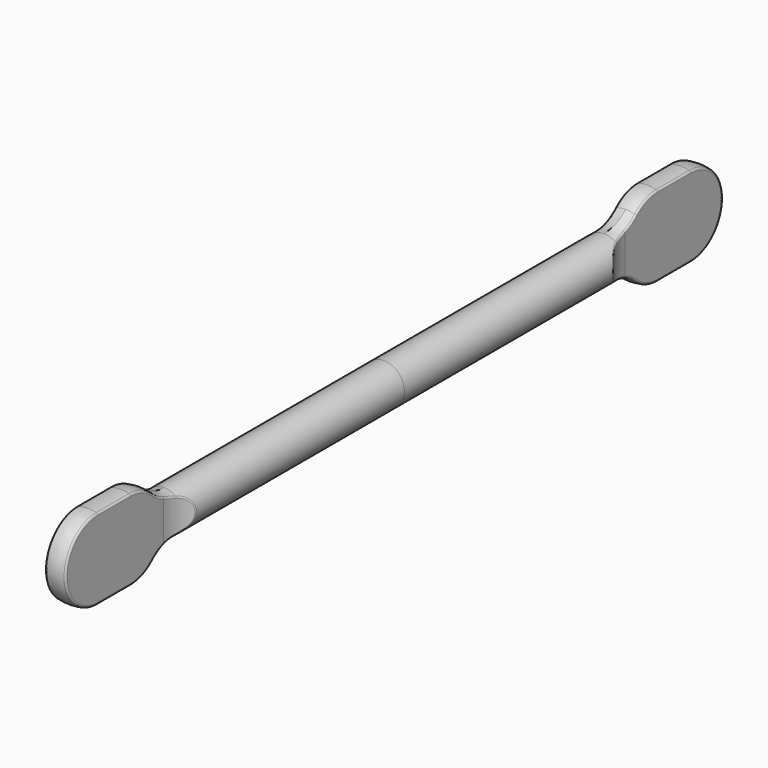
from build123d import *

# Parameters (mm, degrees)
F2_R          = 5
F4_DEPTH      = 5.001
F4_DEPTH_BACK = 5.001
F7_R          = 0.25


with BuildPart() as f1:
    # F0 (on Right) → F1 (revolve)
    with BuildSketch(Plane.YZ):
        with BuildLine():
            Line((35.6698729811, 2.5), (0, 2.5))
            Line((0, 2.5), (0, 0))
            Line((0, 0), (50, 0))
            ThreePointArc((50, 0), (48.5355339059, 3.5355339059), (45, 5))
            Line((45, 5), (40, 5))
            ThreePointArc((40, 5), (37.5, 4.3301270189), (35.6698729811, 2.5))
        make_face()
    revolve(axis=Axis((0, 25, 0), (0, -1, 0)))

    # F2
    f2_edges = [f1.edges().sort_by_distance(p)[0] for p in [
        (0, 35.669873, -2.5),
    ]]
    fillet(f2_edges, radius=F2_R)


with BuildPart() as f4:
    # F3 (on Top) → F4 (new body, two sides)
    with BuildSketch(Plane.XY) as f4_sk:
        with BuildLine():
            Line((-25, 75), (-25, 30))
            Line((-25, 30), (-6.25, 30))
            ThreePointArc((-6.25, 30), (-2.7144660941, 31.4644660941), (-1.25, 35))
            Line((-1.25, 35), (-1.25, 75))
            Line((-1.25, 75), (-25, 75))
        make_face()
    extrude(amount=-F4_DEPTH)
    extrude(f4_sk.sketch, amount=F4_DEPTH_BACK)


with BuildPart() as f5_1:
    # F5: instance of F4
    add(f4.part.mirror(Plane.YZ))


with BuildPart() as f1_1:
    add(f1.part)

    # F6: cut F4, F5_1
    add(f4.part, mode=Mode.SUBTRACT)
    add(f5_1.part, mode=Mode.SUBTRACT)

    # F7
    f7_edges = [f1_1.edges().sort_by_distance(p)[0] for p in [
        (-1.25, 49.841229, 0),
        (1.25, 49.841229, 0),
    ]]
    fillet(f7_edges, radius=F7_R)

    # F8: F1 across plane


with BuildPart() as f1_2:
    add(f1_1.part)
    add(f1_1.part.mirror(Plane.XZ))


solid = f1_2.part
